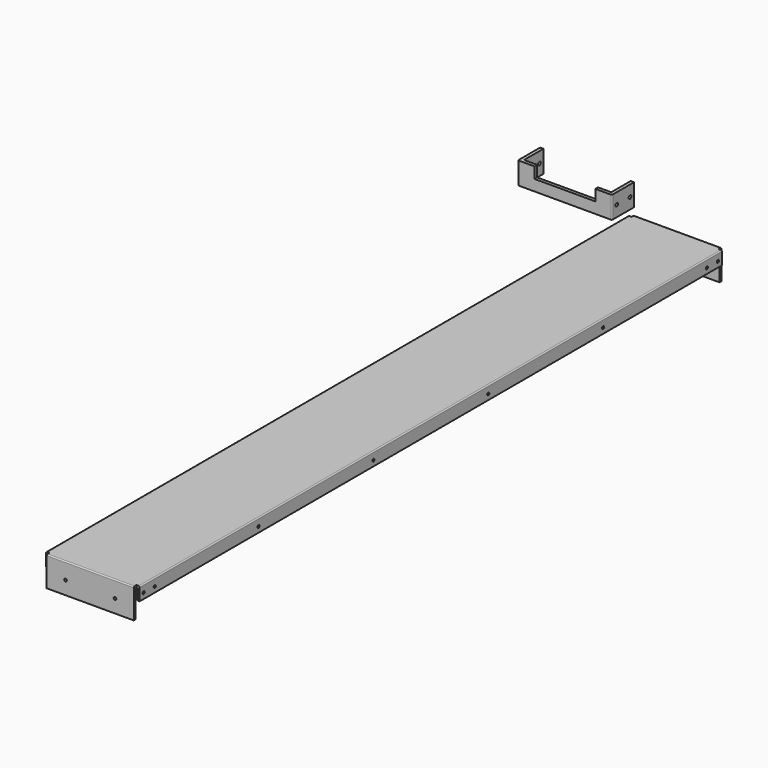
from build123d import *

# Parameters (mm, degrees)
F0_W      = 84.8
F0_H      = 665
F1_DEPTH  = 2
F2_W      = 3
F2_H      = 3
F3_DEPTH  = 2
F4_W      = 78.8
F4_H      = 2
F5_DEPTH  = 25
F4_W_2    = 2
F4_H_2    = 659
F6_DEPTH  = 10
F7_R      = 1
F8_R      = 1.2
F9_DEPTH  = 665.001
F10_R     = 1.2
F11_DEPTH = 84.801
F12_W     = 79
F12_H     = 3
F13_DEPTH = 20
F14_R     = 1.5
F15_DEPTH = 177.0208022366
F16_R     = 0.99999
F17_W     = 55
F17_H     = 10
F18_DEPTH = 3


# Not quite as in the source:
# - a fillet or chamfer is up to 0.001 mm smaller than in the source, because OpenCascade refuses the exact size


with BuildPart() as f1:
    # F0 (on Top) → F1 (new body)
    with BuildSketch(Plane.XY):
        Rectangle(F0_W, F0_H)
    extrude(amount=F1_DEPTH)

    # F2 (on face) → F3 (cut)
    with BuildSketch(Plane.XY.offset(2)):
        with Locations((-40.9, 331)):
            Rectangle(F2_W, F2_H)
        with Locations((40.9, 331)):
            Rectangle(F2_W, F2_H)
        with Locations((40.9, -331)):
            Rectangle(F2_W, F2_H)
        with Locations((-40.9, -331)):
            Rectangle(F2_W, F2_H)
    extrude(amount=-F3_DEPTH, mode=Mode.SUBTRACT)

    # F4 (on face) → F5 (join)
    with BuildSketch(Plane(origin=(0, 0, 0), x_dir=(1, 0, 0), z_dir=(0, 0, -1))):
        with Locations((0, 331.5)):
            Rectangle(F4_W, F4_H)
        with Locations((0, -331.5)):
            Rectangle(F4_W, F4_H)
    extrude(amount=F5_DEPTH)

    # F4 (on face) → F6 (join)
    with BuildSketch(Plane(origin=(0, 0, 0), x_dir=(1, 0, 0), z_dir=(0, 0, -1))):
        with Locations((-41.4, 0)):
            Rectangle(F4_W_2, F4_H_2)
        with Locations((41.4, 0)):
            Rectangle(F4_W_2, F4_H_2)
    extrude(amount=F6_DEPTH)

    # F7
    f7_edges = [f1.edges().sort_by_distance(p)[0] for p in [
        (0, 332.5, 2),
        (-42.4, 0, 2),
        (0, 330.5, 0),
        (42.4, 0, 2),
        (0, -332.5, 2),
        (0, -330.5, 0),
    ]]
    fillet(f7_edges, radius=F7_R)

    # F8 (on face) → F9 (cut, through all)
    with BuildSketch(Plane(origin=(0, 332.5, 0), x_dir=(-1, 0, 0), z_dir=(0, 1, 0))):
        with Locations((-22.4, -13)):
            Circle(F8_R)
        with Locations((22.4, -13)):
            Circle(F8_R)
    extrude(amount=-F9_DEPTH, mode=Mode.SUBTRACT)

    # F10 (on face) → F11 (cut, through all)
    with BuildSketch(Plane.YZ.offset(42.4)):
        with Locations((325, -5)):
            Circle(F10_R)
        with Locations((195, -5)):
            Circle(F10_R)
        with Locations((65, -5)):
            Circle(F10_R)
        with Locations((-65, -5)):
            Circle(F10_R)
        with Locations((-195, -5)):
            Circle(F10_R)
        with Locations((-325, -5)):
            Circle(F10_R)
        with Locations((312.5, -5)):
            Circle(F10_R)
        with Locations((-312.5, -5)):
            Circle(F10_R)
    extrude(amount=-F11_DEPTH, mode=Mode.SUBTRACT)


with BuildPart() as f13:
    # F12 (on Top) → F13 (new body)
    with BuildSketch(Plane.XY):
        with Locations((-92.1198022366, 321.4922089577)):
            Rectangle(F12_W, F12_H)
        Polygon((-131.6198022366, 319.9922089577), (-131.6198022366, 322.9922089577), (-131.6198022366, 344.9922089577), (-134.6198022366, 344.9922089577), (-134.6198022366, 319.9922089577), align=None)
        Polygon((-52.6198022366, 344.9922089577), (-52.6198022366, 322.9922089577), (-52.6198022366, 319.9922089577), (-49.6198022366, 319.9922089577), (-49.6198022366, 344.9922089577), align=None)
    extrude(amount=F13_DEPTH)

    # F14 (on face) → F15 (cut, through all)
    with BuildSketch(Plane(origin=(-134.6198022366, 0, 0), x_dir=(0, -1, 0), z_dir=(-1, 0, 0))):
        with Locations((-325.4922089577, 10)):
            Circle(F14_R)
        with Locations((-340.4922089577, 10)):
            Circle(F14_R)
    extrude(amount=-F15_DEPTH, mode=Mode.SUBTRACT)

    # F16 (radius 1 in the source; OpenCascade refuses exactly that, so slightly less here)
    f16_edges = [f13.edges().sort_by_distance(p)[0] for p in [
        (-49.619802, 319.992209, 10),
        (-52.619802, 322.992209, 10),
        (-134.619802, 319.992209, 10),
        (-131.619802, 322.992209, 10),
    ]]
    fillet(f16_edges, radius=F16_R)

    # F17 (on face) → F18 (cut)
    with BuildSketch(Plane.XZ.offset(-319.9922089577)):
        with Locations((-92.1198022366, 15)):
            Rectangle(F17_W, F17_H)
    extrude(amount=-F18_DEPTH, mode=Mode.SUBTRACT)


solid = Compound([f1.part, f13.part])
